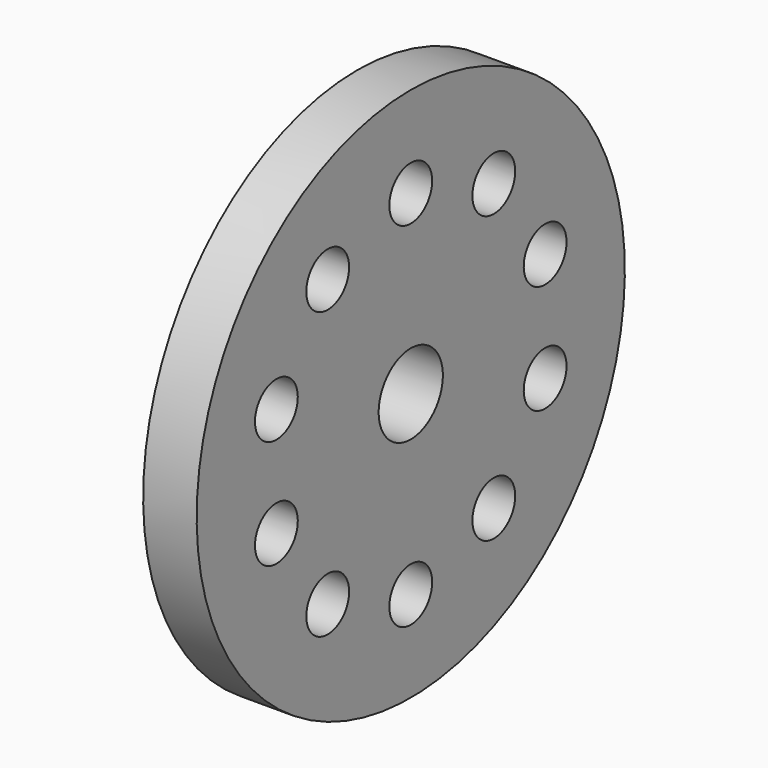
from build123d import *

# Parameters (mm, degrees)
F3_D            = 12.7
F3_COPIES_COUNT = 10


# Not quite as in the source:
# - a pattern or mirror of a feature is missing from the dataset's text; its kind, count and spacing are read off the source's solid


with BuildPart() as f1:
    # F0 (on Front) → F1 (revolve)
    with BuildSketch(Plane.XZ):
        Polygon((12.7, 0), (0, 0), (0, -38.1), (-12.7, -38.1), (-12.7, -53.975), (12.7, -53.975), align=None)
    revolve(axis=Axis((40.5070465058, 0, -63.5), (1, 0, 0)))

    # F3 (through all)
    with Locations(Plane(origin=(0, 0, 0), x_dir=(0, -1, 0), z_dir=(-1, 0, 0))):
        with Locations((0, -21.59)):
            f3 = Hole(F3_D / 2)

    # F3_copies: F3 ×10 about axis
    f3_copies_axis = Axis((0, 0, -63.5), (1, 0, 0))
    for i in range(1, F3_COPIES_COUNT):
        add(f3.rotate(f3_copies_axis, i * 360 / F3_COPIES_COUNT), mode=Mode.SUBTRACT)


solid = f1.part
